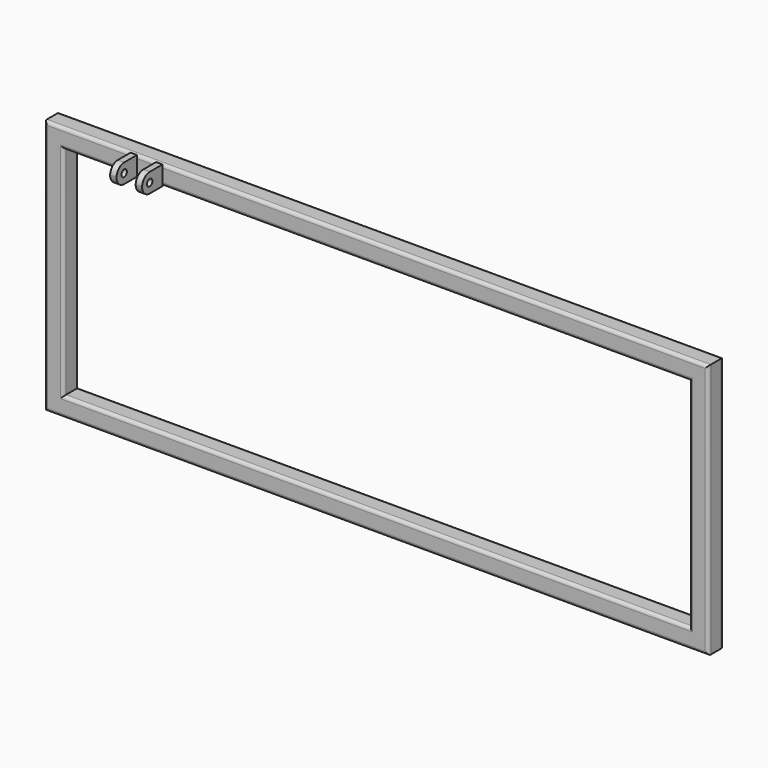
from build123d import *

# Parameters (mm, degrees)
F0_W     = 1320.8
F0_H     = 508
F0_W_2   = 1244.6
F0_H_2   = 431.8
F1_DEPTH = 38.1
F2_R     = 6.35
F3_W     = 12.7
F3_H     = 38.1
F4_DEPTH = 50.8
F5_R     = 19.04999
F7_D     = 13.49248


# Not quite as in the source:
# - a fillet or chamfer is up to 0.001 mm smaller than in the source, because OpenCascade refuses the exact size


with BuildPart() as f1:
    # F0 (on Front) → F1 (new body)
    with BuildSketch(Plane.XZ):
        Rectangle(F0_W, F0_H)
        Rectangle(F0_W_2, F0_H_2, mode=Mode.SUBTRACT)
    extrude(amount=F1_DEPTH)

    # F2
    f2_edges = [f1.edges().sort_by_distance(p)[0] for p in [
        (0, -38.1, 254),
        (-660.4, -38.1, 0),
        (0, -38.1, -254),
        (660.4, -38.1, 0),
        (-622.3, -38.1, 0),
        (0, -38.1, 215.9),
        (622.3, -38.1, 0),
        (0, -38.1, -215.9),
        (0, 0, 254),
        (-660.4, 0, 0),
        (0, 0, -254),
        (660.4, 0, 0),
        (-622.3, 0, 0),
        (0, 0, 215.9),
        (622.3, 0, 0),
        (0, 0, -215.9),
    ]]
    fillet(f2_edges, radius=F2_R)


with BuildPart() as f4:
    # F3 (on face) → F4 (new body)
    with BuildSketch(Plane.XZ.offset(38.1)):
        with Locations((-482.6, 234.95)):
            Rectangle(F3_W, F3_H)
    extrude(amount=F4_DEPTH)

    # F5 (radius 19.05 in the source; OpenCascade refuses exactly that, so slightly less here)
    f5_edges = [f4.edges().sort_by_distance(p)[0] for p in [
        (-482.6, -88.9, 254),
        (-482.6, -88.9, 215.9),
    ]]
    fillet(f5_edges, radius=F5_R)

    # F7 (through all)
    with Locations(Plane.YZ.offset(-476.25)):
        with Locations((-69.85, 234.95)):
            Hole(F7_D / 2)


with BuildPart() as f9_1:
    # F9: instance of F4
    add(f4.part.mirror(Plane(origin=(-457.2, -60.9330603651, 234.95), x_dir=(0, 1, 0), z_dir=(1, 0, 0))))


solid = Compound([f1.part, f4.part, f9_1.part])
